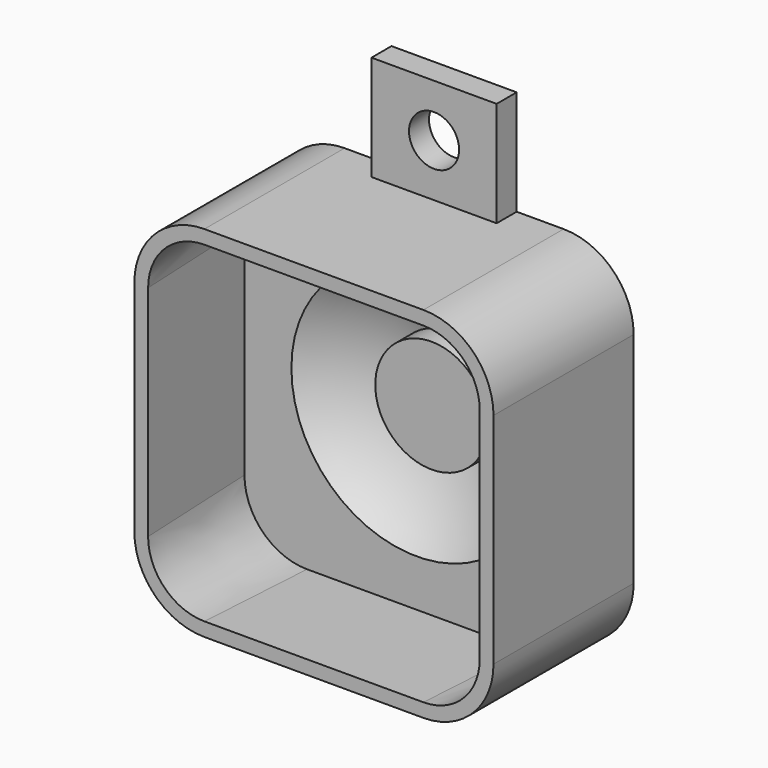
from build123d import *

# Parameters (mm, degrees)
F0_R      = 20
F0_R_2    = 9
F2_DEPTH  = 20.5
F3_SIZE2  = 20.49999
F3_SIZE   = 0.99999
F5_DEPTH  = 3.5
F7_DEPTH  = 28
F9_W      = 20
F9_H      = 8.2
F9_H_2    = 16.8
F9_R      = 4
F10_DEPTH = 4


# Not quite as in the source:
# - a fillet or chamfer is up to 0.001 mm smaller than in the source, because OpenCascade refuses the exact size
# - a feature names something its author has since deleted; it is built from what else it names


with BuildPart() as f2:
    # F0 (on Front) → F2 (new body)
    with BuildSketch(Plane.XZ):
        with BuildLine():
            Line((-17.5, -27.5), (17.5, -27.5))
            ThreePointArc((17.5, -27.5), (24.5710678119, -24.5710678119), (27.5, -17.5))
            Line((27.5, -17.5), (27.5, 17.5))
            ThreePointArc((27.5, 17.5), (24.5710678119, 24.5710678119), (17.5, 27.5))
            Line((17.5, 27.5), (-17.5, 27.5))
            ThreePointArc((-17.5, 27.5), (-24.5710678119, 24.5710678119), (-27.5, 17.5))
            Line((-27.5, 17.5), (-27.5, -17.5))
            ThreePointArc((-27.5, -17.5), (-24.5710678119, -24.5710678119), (-17.5, -27.5))
        make_face()
        with BuildLine():
            ThreePointArc((17.5, 26.5), (23.8639610307, 23.8639610307), (26.5, 17.5))
            Line((26.5, 17.5), (26.5, -17.5))
            ThreePointArc((26.5, -17.5), (23.8639610307, -23.8639610307), (17.5, -26.5))
            Line((17.5, -26.5), (-17.5, -26.5))
            ThreePointArc((-17.5, -26.5), (-23.8639610307, -23.8639610307), (-26.5, -17.5))
            Line((-26.5, -17.5), (-26.5, 17.5))
            ThreePointArc((-26.5, 17.5), (-23.8639610307, 23.8639610307), (-17.5, 26.5))
            Line((-17.5, 26.5), (17.5, 26.5))
        make_face(mode=Mode.SUBTRACT)
        with BuildLine():
            Line((26.5, -17.5), (26.5, 17.5))
            ThreePointArc((26.5, 17.5), (23.8639610307, 23.8639610307), (17.5, 26.5))
            Line((17.5, 26.5), (-17.5, 26.5))
            ThreePointArc((-17.5, 26.5), (-23.8639610307, 23.8639610307), (-26.5, 17.5))
            Line((-26.5, 17.5), (-26.5, -17.5))
            ThreePointArc((-26.5, -17.5), (-23.8639610307, -23.8639610307), (-17.5, -26.5))
            Line((-17.5, -26.5), (17.5, -26.5))
            ThreePointArc((17.5, -26.5), (23.8639610307, -23.8639610307), (26.5, -17.5))
        make_face()
        with BuildLine():
            ThreePointArc((17.5, 25.5), (23.1568542495, 23.1568542495), (25.5, 17.5))
            Line((25.5, 17.5), (25.5, -17.5))
            ThreePointArc((25.5, -17.5), (23.1568542495, -23.1568542495), (17.5, -25.5))
            Line((17.5, -25.5), (-17.5, -25.5))
            ThreePointArc((-17.5, -25.5), (-23.1568542495, -23.1568542495), (-25.5, -17.5))
            Line((-25.5, -17.5), (-25.5, 17.5))
            ThreePointArc((-25.5, 17.5), (-23.1568542495, 23.1568542495), (-17.5, 25.5))
            Line((-17.5, 25.5), (17.5, 25.5))
        make_face(mode=Mode.SUBTRACT)
        with BuildLine():
            Line((25.5, -17.5), (25.5, 17.5))
            ThreePointArc((25.5, 17.5), (23.1568542495, 23.1568542495), (17.5, 25.5))
            Line((17.5, 25.5), (-17.5, 25.5))
            ThreePointArc((-17.5, 25.5), (-23.1568542495, 23.1568542495), (-25.5, 17.5))
            Line((-25.5, 17.5), (-25.5, -17.5))
            ThreePointArc((-25.5, -17.5), (-23.1568542495, -23.1568542495), (-17.5, -25.5))
            Line((-17.5, -25.5), (17.5, -25.5))
            ThreePointArc((17.5, -25.5), (23.1568542495, -23.1568542495), (25.5, -17.5))
        make_face()
        Circle(F0_R, mode=Mode.SUBTRACT)
        Circle(F0_R)
        Circle(F0_R_2, mode=Mode.SUBTRACT)
        Circle(F0_R_2)
    extrude(amount=F2_DEPTH)

    # F3 (size 1 and 20.5 in the source; OpenCascade refuses exactly that, so slightly less here)
    f3_edges = [f2.edges().sort_by_distance(p)[0] for p in [
        (0, -20.5, -27.5),
        (24.571068, -20.5, -24.571068),
        (27.5, -20.5, 0),
        (24.571068, -20.5, 24.571068),
        (0, -20.5, 27.5),
        (-24.571068, -20.5, 24.571068),
        (-27.5, -20.5, 0),
        (-24.571068, -20.5, -24.571068),
    ]]
    f3_side = f2.faces().sort_by_distance((0, -20.5, 0))[0]
    chamfer(f3_edges, length=F3_SIZE, length2=F3_SIZE2, reference=f3_side)

    # F1 (on Top) → F4 (revolve)
    with BuildSketch(Plane.XY):
        with BuildLine():
            Line((9, 0), (20, 0))
            ThreePointArc((20, 0), (14.8597611017, 3.8588264798), (9, 6.5))
            Line((9, 6.5), (0, 6.5))
            Line((0, 6.5), (0, 0))
            Line((0, 0), (9, 0))
        make_face()
    revolve(axis=Axis((0, 3.25, 0), (0, 1, 0)))

    # F5 (cut): a face of the model
    f5_faces = [f2.faces().sort_by_distance(p)[0] for p in [
        (0, 6.5, 0),
    ]]
    extrude(f5_faces, amount=-F5_DEPTH, mode=Mode.SUBTRACT)


with BuildPart() as f7:
    # F6 (on face) → F7 (new body)
    with BuildSketch(Plane.XZ.offset(20.5)):
        with BuildLine():
            Line((-28.7, 17.5), (-28.7, -17.5))
            ThreePointArc((-28.7, -17.5), (-25.4195959493, -25.4195959493), (-17.5, -28.7))
            Line((-17.5, -28.7), (17.5, -28.7))
            ThreePointArc((17.5, -28.7), (25.4195959493, -25.4195959493), (28.7, -17.5))
            Line((28.7, -17.5), (28.7, 17.5))
            ThreePointArc((28.7, 17.5), (25.4195959493, 25.4195959493), (17.5, 28.7))
            Line((17.5, 28.7), (-17.5, 28.7))
            ThreePointArc((-17.5, 28.7), (-25.4195959493, 25.4195959493), (-28.7, 17.5))
        make_face()
        with BuildLine():
            Line((17.5, -26.50001), (-17.5, -26.50001))
            ThreePointArc((-17.5, -26.50001), (-23.8639681017, -23.8639681017), (-26.50001, -17.5))
            Line((-26.50001, -17.5), (-26.50001, 17.5))
            ThreePointArc((-26.50001, 17.5), (-23.8639681017, 23.8639681017), (-17.5, 26.50001))
            Line((-17.5, 26.50001), (17.5, 26.50001))
            ThreePointArc((17.5, 26.50001), (23.8639681017, 23.8639681017), (26.50001, 17.5))
            Line((26.50001, 17.5), (26.50001, -17.5))
            ThreePointArc((26.50001, -17.5), (23.8639681017, -23.8639681017), (17.5, -26.50001))
        make_face(mode=Mode.SUBTRACT)
        with BuildLine():
            ThreePointArc((-26.50001, -17.5), (-23.8639681017, -23.8639681017), (-17.5, -26.50001))
            Line((-17.5, -26.50001), (17.5, -26.50001))
            ThreePointArc((17.5, -26.50001), (23.8639681017, -23.8639681017), (26.50001, -17.5))
            Line((26.50001, -17.5), (26.50001, 17.5))
            ThreePointArc((26.50001, 17.5), (23.8639681017, 23.8639681017), (17.5, 26.50001))
            Line((17.5, 26.50001), (-17.5, 26.50001))
            ThreePointArc((-17.5, 26.50001), (-23.8639681017, 23.8639681017), (-26.50001, 17.5))
            Line((-26.50001, 17.5), (-26.50001, -17.5))
        make_face()
    extrude(amount=-F7_DEPTH)

    # F8: cut F2
    add(f2.part, mode=Mode.SUBTRACT)

    # F9 (on face) → F10 (join)
    with BuildSketch(Plane(origin=(0, 7.5, 0), x_dir=(-1, 0, 0), z_dir=(0, 1, 0))):
        with Locations((0, 24.6)):
            Rectangle(F9_W, F9_H)
        with Locations((0, 37.1)):
            Rectangle(F9_W, F9_H_2)
        with Locations((0, 37.1)):
            Circle(F9_R, mode=Mode.SUBTRACT)
    extrude(amount=-F10_DEPTH)


solid = f7.part
